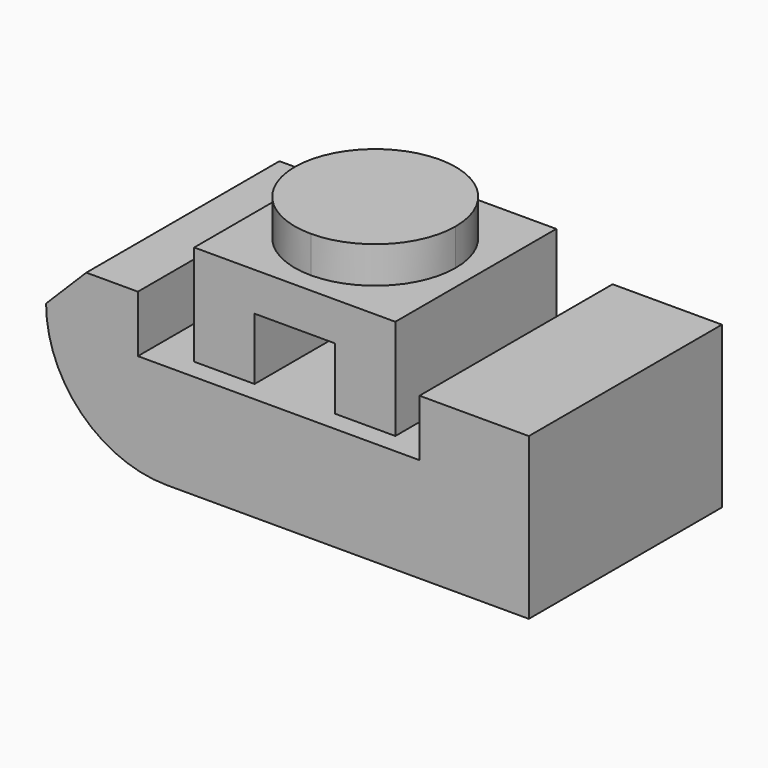
from build123d import *

# Parameters (mm, degrees)
F1_DEPTH = 30
F2_DEPTH = 25
F0_W     = 40
F0_H     = 9.0879101008
F3_DEPTH = 20
F4_R     = 30
F5_SIZE  = 9.99999
F6_R     = 19.99999


# Not quite as in the source:
# - a fillet or chamfer is up to 0.001 mm smaller than in the source, because OpenCascade refuses the exact size


with BuildPart() as f1:
    # F0 (on Front) → F1 (new body, symmetric)
    with BuildSketch(Plane.XZ):
        Polygon((-57.820021317, -12.9469532817), (-35, -12.9469532817), (-35, 12.9469532817), (-35, 27.0530467183), (-57.820021317, 27.0530467183), align=None)
        Polygon((-35, -12.9469532817), (35, -12.9469532817), (35, 12.9469532817), (25, 12.9469532817), (10, 12.9469532817), (-10, 12.9469532817), (-25, 12.9469532817), (-35, 12.9469532817), align=None)
        Polygon((35, 12.9469532817), (35, -12.9469532817), (62.179978683, -12.9469532817), (62.179978683, 27.0530467183), (35, 27.0530467183), align=None)
    extrude(amount=F1_DEPTH, both=True)

    # F0 (on Front) → F2 (join, symmetric)
    with BuildSketch(Plane.XZ):
        Polygon((10, 12.9469532817), (25, 12.9469532817), (25, 37.9469532817), (20, 37.9469532817), (-20, 37.9469532817), (-25, 37.9469532817), (-25, 12.9469532817), (-10, 12.9469532817), (-10, 28.3428579569), (10, 28.3428579569), align=None)
    extrude(amount=F2_DEPTH, both=True)

    # F0 (on Front) → F3 (join, symmetric)
    with BuildSketch(Plane.XZ):
        with Locations((0, 42.4909083322)):
            Rectangle(F0_W, F0_H)
    extrude(amount=F3_DEPTH, both=True)

    # F4
    f4_edges = [f1.edges().sort_by_distance(p)[0] for p in [
        (-57.820021, 0, -12.946953),
    ]]
    fillet(f4_edges, radius=F4_R)

    # F5 (size 10 in the source; OpenCascade refuses exactly that, so slightly less here)
    f5_edges = [f1.edges().sort_by_distance(p)[0] for p in [
        (-57.820021, 0, 27.053047),
    ]]
    chamfer(f5_edges, length=F5_SIZE)

    # F6 (radius 20 in the source; OpenCascade refuses exactly that, so slightly less here)
    f6_edges = [f1.edges().sort_by_distance(p)[0] for p in [
        (20, -20, 42.490908),
        (20, 20, 42.490908),
        (-20, -20, 42.490908),
        (-20, 20, 42.490908),
    ]]
    fillet(f6_edges, radius=F6_R)


solid = f1.part
